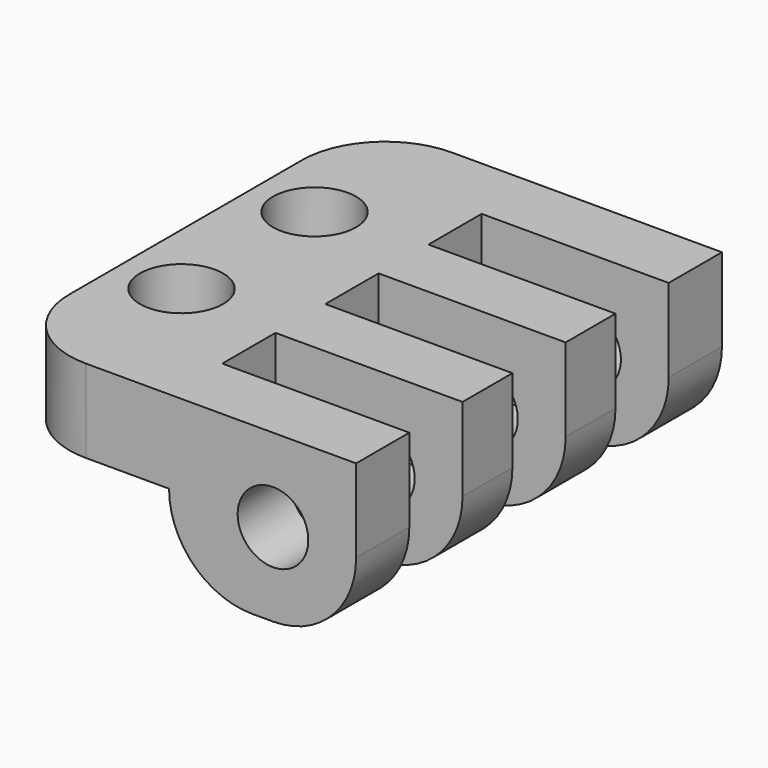
from build123d import *

# Parameters (mm, degrees)
F0_W     = 7
F0_H     = 18
F0_R     = 2
F0_W_2   = 10
F1_DEPTH = 8
F3_D     = 3.4
F4_W     = 9
F4_H     = 3.2
F5_DEPTH = 25
F6_DEPTH = 2
F7_DEPTH = 2
F8_R     = 2
F9_DEPTH = 4
F10_R    = 3.99999


# Not quite as in the source:
# - a fillet or chamfer is up to 0.001 mm smaller than in the source, because OpenCascade refuses the exact size


with BuildPart() as f1:
    # F0 (on Top) → F1 (new body)
    with BuildSketch(Plane.XY):
        with Locations((-1.6666666667, 0)):
            Rectangle(F0_W, F0_H)
        with Locations((-2.1666666667, -4)):
            Circle(F0_R, mode=Mode.SUBTRACT)
        with Locations((-2.1666666667, 4)):
            Circle(F0_R, mode=Mode.SUBTRACT)
        with Locations((6.8333333333, 0)):
            Rectangle(F0_W_2, F0_H)
    extrude(amount=F1_DEPTH)

    # F3 (through all)
    with Locations(Plane.XZ.offset(9)):
        with Locations((7.8333333333, 4)):
            Hole(F3_D / 2)

    # F4 (on face) → F5 (cut)
    with BuildSketch(Plane.XY.offset(8)):
        with Locations((7.3333333333, 6.2)):
            Rectangle(F4_W, F4_H)
        with Locations((7.3333333333, 0)):
            Rectangle(F4_W, F4_H)
        with Locations((7.3333333333, -6.2)):
            Rectangle(F4_W, F4_H)
    extrude(amount=-F5_DEPTH, mode=Mode.SUBTRACT)

    # F6 (add): a face of the model
    f6_faces = [f1.faces().sort_by_distance(p)[0] for p in [
        (3.0114285443, -9, 4),
    ]]
    extrude(f6_faces, amount=F6_DEPTH)

    # F7 (add): a face of the model
    f7_faces = [f1.faces().sort_by_distance(p)[0] for p in [
        (3.0114285443, 9, 4),
    ]]
    extrude(f7_faces, amount=F7_DEPTH)

    # F8 (on face) → F9 (cut)
    with BuildSketch(Plane(origin=(0, 0, 0), x_dir=(1, 0, 0), z_dir=(0, 0, -1))):
        Polygon((2.8333333333, 7.8), (2.8333333333, 11), (-5.1666666667, 11), (-5.1666666667, -11), (2.8333333333, -11), (2.8333333333, -7.8), (2.8333333333, -4.6), (2.8333333333, -1.6), (2.8333333333, 1.6), (2.8333333333, 4.6), align=None)
        with Locations((-2.1666666667, -4)):
            Circle(F8_R, mode=Mode.SUBTRACT)
        with Locations((-2.1666666667, 4)):
            Circle(F8_R, mode=Mode.SUBTRACT)
    extrude(amount=-F9_DEPTH, mode=Mode.SUBTRACT)

    # F10 (radius 4 in the source; OpenCascade refuses exactly that, so slightly less here)
    f10_edges = [f1.edges().sort_by_distance(p)[0] for p in [
        (-5.166667, -11, 6),
        (-5.166667, 11, 6),
        (2.833333, -9.4, 0),
        (2.833333, -3.1, 0),
        (2.833333, 3.1, 0),
        (2.833333, 9.4, 0),
        (11.833333, -9.4, 0),
        (11.833333, -3.1, 0),
        (11.833333, 3.1, 0),
        (11.833333, 9.4, 0),
    ]]
    fillet(f10_edges, radius=F10_R)


solid = f1.part
